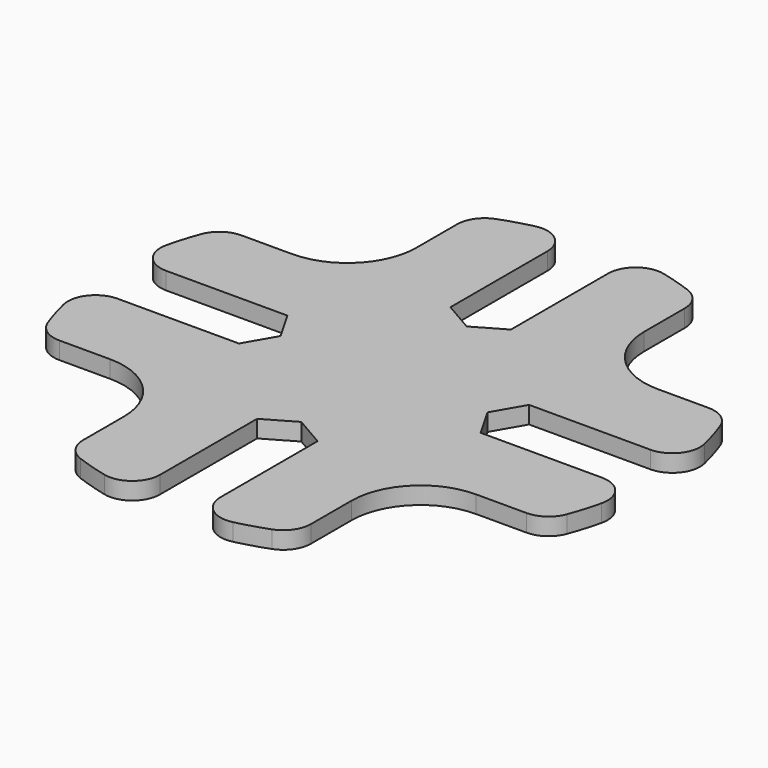
from build123d import *

# Parameters (mm, degrees)
F1_DEPTH = 1.5875
F2_R     = 6.35
F3_R     = 2.54


# Not quite as in the source:
# - a feature names something its author has since deleted; it is built from what else it names


with BuildPart() as f1:
    # F0 (on Top) → F1 (new body)
    with BuildSketch(Plane.XY):
        with BuildLine():
            Line((14.3039512166, 2.778125), (25.2476141741, 2.778125))
            ThreePointArc((25.2476141741, 2.778125), (24.5012506268, 6.6969185243), (23.1505208253, 10.4505208253))
            Line((23.1505208253, 10.4505208253), (10.4505208253, 10.4505208253))
            Line((10.4505208253, 10.4505208253), (10.4505208253, 23.1505208253))
            ThreePointArc((10.4505208253, 23.1505208253), (6.6969185243, 24.5012506268), (2.778125, 25.2476141741))
            Line((2.778125, 25.2476141741), (2.778125, 14.3039512166))
            Line((2.778125, 14.3039512166), (2.778125, 11.0960487834))
            Line((2.778125, 11.0960487834), (0, 9.4920975668))
            Line((0, 9.4920975668), (-2.778125, 11.0960487834))
            Line((-2.778125, 11.0960487834), (-2.778125, 14.3039512166))
            Line((-2.778125, 14.3039512166), (-2.778125, 25.2476141741))
            ThreePointArc((-2.778125, 25.2476141741), (-6.6969185243, 24.5012506268), (-10.4505208253, 23.1505208253))
            Line((-10.4505208253, 23.1505208253), (-10.4505208253, 10.4505208253))
            Line((-10.4505208253, 10.4505208253), (-23.1505208253, 10.4505208253))
            ThreePointArc((-23.1505208253, 10.4505208253), (-24.5012506268, 6.6969185243), (-25.2476141741, 2.778125))
            Line((-25.2476141741, 2.778125), (-14.3039512166, 2.778125))
            Line((-14.3039512166, 2.778125), (-11.0960487834, 2.778125))
            Line((-11.0960487834, 2.778125), (-9.4920975668, 0))
            Line((-9.4920975668, 0), (-11.0960487834, -2.778125))
            Line((-11.0960487834, -2.778125), (-14.3039512166, -2.778125))
            Line((-14.3039512166, -2.778125), (-25.2476141741, -2.778125))
            ThreePointArc((-25.2476141741, -2.778125), (-24.5012506268, -6.6969185243), (-23.1505208253, -10.4505208253))
            Line((-23.1505208253, -10.4505208253), (-10.4505208253, -10.4505208253))
            Line((-10.4505208253, -10.4505208253), (-10.4505208253, -23.1505208253))
            ThreePointArc((-10.4505208253, -23.1505208253), (-6.6969185243, -24.5012506268), (-2.778125, -25.2476141741))
            Line((-2.778125, -25.2476141741), (-2.778125, -14.3039512166))
            Line((-2.778125, -14.3039512166), (-2.778125, -11.0960487834))
            Line((-2.778125, -11.0960487834), (0, -9.4920975668))
            Line((0, -9.4920975668), (2.778125, -11.0960487834))
            Line((2.778125, -11.0960487834), (2.778125, -14.3039512166))
            Line((2.778125, -14.3039512166), (2.778125, -25.2476141741))
            ThreePointArc((2.778125, -25.2476141741), (6.6969185243, -24.5012506268), (10.4505208253, -23.1505208253))
            Line((10.4505208253, -23.1505208253), (10.4505208253, -10.4505208253))
            Line((10.4505208253, -10.4505208253), (23.1505208253, -10.4505208253))
            ThreePointArc((23.1505208253, -10.4505208253), (24.5012506268, -6.6969185243), (25.2476141741, -2.778125))
            Line((25.2476141741, -2.778125), (14.3039512166, -2.778125))
            Line((14.3039512166, -2.778125), (11.0960487834, -2.778125))
            Line((11.0960487834, -2.778125), (9.4920975668, 0))
            Line((9.4920975668, 0), (11.0960487834, 2.778125))
            Line((11.0960487834, 2.778125), (14.3039512166, 2.778125))
        make_face()
    extrude(amount=F1_DEPTH)

    # F2
    f2_edges = [f1.edges().sort_by_distance(p)[0] for p in [
        (-10.450521, -10.450521, 0.79375),
        (10.450521, -10.450521, 0.79375),
        (10.450521, 10.450521, 0.79375),
        (-10.450521, 10.450521, 0.79375),
    ]]
    fillet(f2_edges, radius=F2_R)

    # F3
    f3_edges = [f1.edges().sort_by_distance(p)[0] for p in [
        (2.778125, 25.247614, 0.79375),
        (-2.778125, 25.247614, 0.79375),
        (25.247614, 2.778125, 0.79375),
        (25.247614, -2.778125, 0.79375),
        (2.778125, -25.247614, 0.79375),
        (-2.778125, -25.247614, 0.79375),
        (-25.247614, -2.778125, 0.79375),
        (-25.247614, 2.778125, 0.79375),
        (23.150521, 10.450521, 0.79375),
        (10.450521, -23.150521, 0.79375),
        (-10.450521, -23.150521, 0.79375),
        (-23.150521, -10.450521, 0.79375),
        (-23.150521, 10.450521, 0.79375),
        (-10.450521, 23.150521, 0.79375),
        (10.450521, 23.150521, 0.79375),
        (23.150521, -10.450521, 0.79375),
    ]]
    fillet(f3_edges, radius=F3_R)


solid = f1.part
